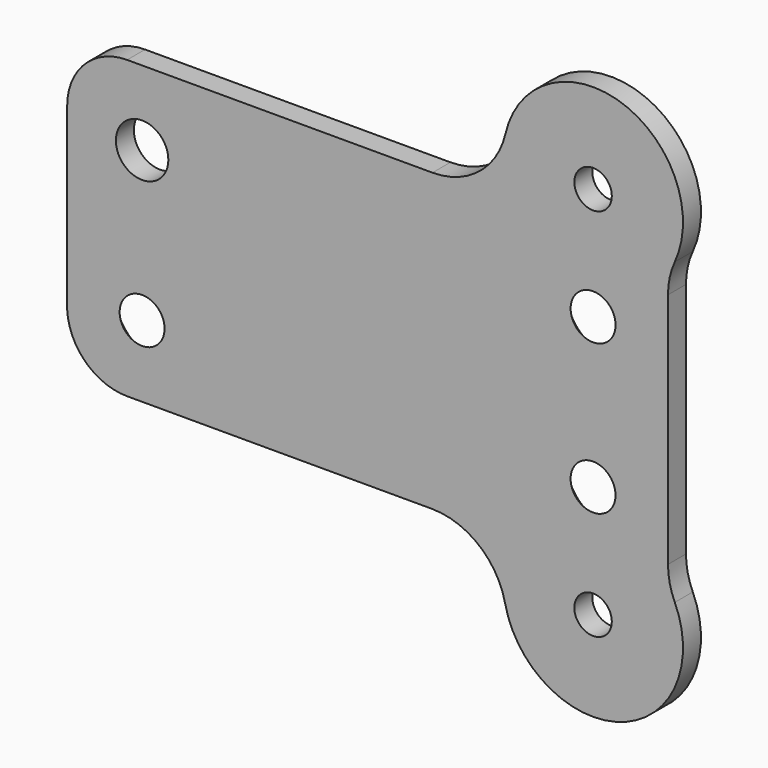
from build123d import *

# Parameters (mm, degrees)
F0_R     = 2.5
F0_R_2   = 3.5
F1_DEPTH = 3


# Not quite as in the source:
# - a fillet or chamfer that OpenCascade refuses, or shapes differently, is made with other operations: its cross-section is extruded or revolved along the edge and cut away or added


with BuildPart() as f1:
    # F0 (on Front) → F1 (new body)
    with BuildSketch(Plane.XZ):
        with BuildLine():
            ThreePointArc((8.6618165432, -19.5581924259), (14.9578845034, -21.7890529471), (18.4448225733, -27.4862867778))
            ThreePointArc((18.4448225733, -27.4862867778), (33.9501260505, -36.3938374492), (41.0935207185, -20.0008265146))
            ThreePointArc((41.0935207185, -20.0008265146), (40.4143456003, -17.9668557736), (40.1844298095, -15.8348486101))
            Line((40.1844298095, -15.8348486101), (40.1844298095, 15.8348486101))
            ThreePointArc((40.1844298095, 15.8348486101), (40.4143456003, 17.9668557736), (41.0935207185, 20.0008265146))
            ThreePointArc((41.0935207185, 20.0008265146), (34.0564016131, 36.3581615745), (18.4933227899, 27.7051832948))
            ThreePointArc((18.4933227899, 27.7051832948), (14.9739484465, 22.1318851219), (8.750733607, 19.9595027072))
            Line((8.750733607, 19.9595027072), (-32, 19.9595027072))
            ThreePointArc((-32, 19.9595027072), (-37.6568542495, 17.6163569566), (-40, 11.9595027072))
            Line((-40, 11.9595027072), (-40, -12))
            ThreePointArc((-40, -12), (-37.5106423232, -17.3691502038), (-32.0122089369, -19.5581924259))
            Line((-32.0122089369, -19.5581924259), (8.6618165432, -19.5581924259))
        make_face()
        with Locations((-30, -10)):
            Circle(F0_R, mode=Mode.SUBTRACT)
        with Locations((30.1844298095, -25)):
            Circle(F0_R, mode=Mode.SUBTRACT)
        with Locations((30.1844298095, -10)):
            Circle(F0_R, mode=Mode.SUBTRACT)
        with Locations((-30, 10)):
            Circle(F0_R_2, mode=Mode.SUBTRACT)
        with Locations((30.1844298095, 10)):
            Circle(F0_R, mode=Mode.SUBTRACT)
        with Locations((30.1844298095, 25)):
            Circle(F0_R, mode=Mode.SUBTRACT)
    extrude(amount=F1_DEPTH)

    # F2: chamfer of 3.5 on 3 edges, made by hand

    # F2_s1 → F2_t2 (revolve, cut)
    with BuildSketch(Plane.XY.offset(10)):
        Polygon((32.6844298095, -3.5), (36.1844298095, 0), (32.6844298095, 0), align=None)
    revolve(axis=Axis((30.1844298095, 0, 10), (0, -1, 0)), mode=Mode.SUBTRACT)

    # F2_s3 → F2_t4 (revolve, cut)
    with BuildSketch(Plane.XY.offset(-10)):
        Polygon((32.6844298095, -3.5), (36.1844298095, 0), (32.6844298095, 0), align=None)
    revolve(axis=Axis((30.1844298095, 0, -10), (0, -1, 0)), mode=Mode.SUBTRACT)

    # F2_s5 → F2_t6 (revolve, cut)
    with BuildSketch(Plane.XY.offset(-10)):
        Polygon((-27.5, -3.5), (-24, 0), (-27.5, 0), align=None)
    revolve(axis=Axis((-30, 0, -10), (0, -1, 0)), mode=Mode.SUBTRACT)


solid = f1.part
